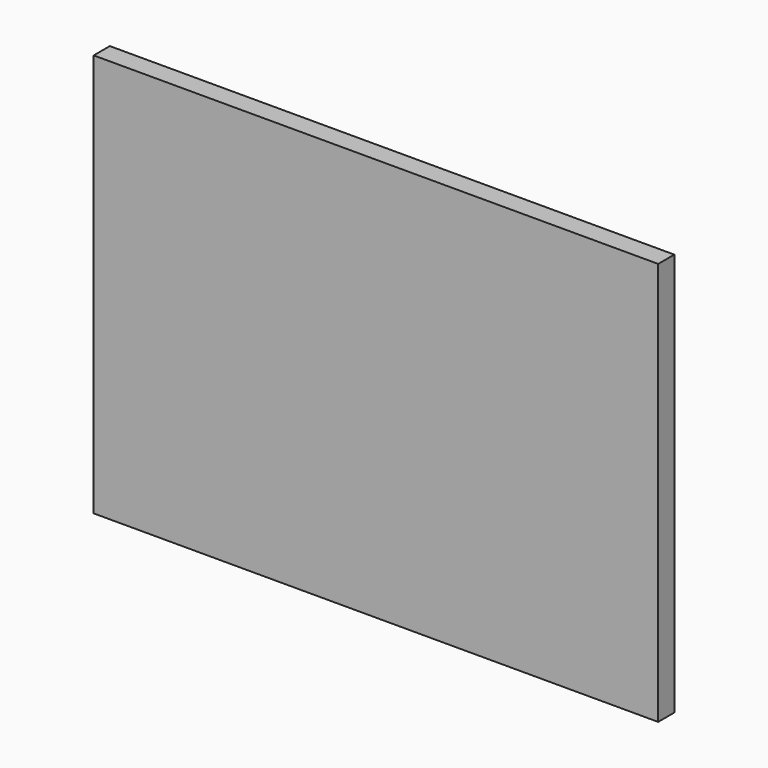
from build123d import *

# Parameters (mm, degrees)
F0_W     = 177.8
F0_H     = 127
F1_DEPTH = 6.35


# Not quite as in the source:
# - a length typed as a fraction of an inch, garbled in the dataset ("3 / 203.2 mm" for 3/8 in), is restored


with BuildPart() as f1:
    # F0 (on Front) → F1 (new body)
    with BuildSketch(Plane.XZ):
        with Locations((88.9, 63.5)):
            Rectangle(F0_W, F0_H)
    extrude(amount=F1_DEPTH)


solid = f1.part
